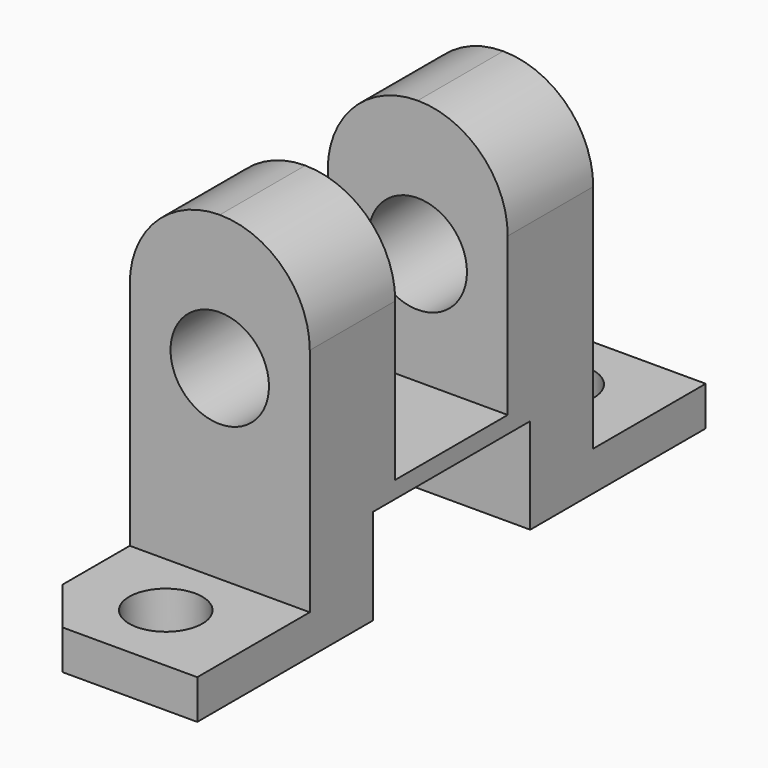
from build123d import *

# Parameters (mm, degrees)
F0_W      = 32
F0_H      = 113
F1_DEPTH  = 20
F2_W      = 32
F2_H      = 25
F3_DEPTH  = 13
F4_W      = 32
F4_H      = 35
F5_DEPTH  = 17
F6_W      = 32
F6_H      = 19
F7_DEPTH  = 44
F8_R      = 16
F9_R      = 15.99999
F10_R     = 16
F11_R     = 15.99999
F12_R     = 6.5
F13_DEPTH = 13
F14_R     = 6.5
F15_DEPTH = 13
F17_DEPTH = 25
F19_DEPTH = 25
F20_R     = 8.75
F21_DEPTH = 100


# Not quite as in the source:
# - a fillet or chamfer is up to 0.001 mm smaller than in the source, because OpenCascade refuses the exact size


with BuildPart() as f1:
    # F0 (on Top) → F1 (new body)
    with BuildSketch(Plane.XY):
        with Locations((-23.4775710851, 33.1401875504)):
            Rectangle(F0_W, F0_H)
    extrude(amount=F1_DEPTH)

    # F2 (on face) → F3 (cut)
    with BuildSketch(Plane.XY.offset(20)):
        with Locations((-23.4775710851, 77.1401875504)):
            Rectangle(F2_W, F2_H)
        with Locations((-23.4775710851, -10.8598124496)):
            Rectangle(F2_W, F2_H)
    extrude(amount=-F3_DEPTH, mode=Mode.SUBTRACT)

    # F4 (on face) → F5 (cut)
    with BuildSketch(Plane(origin=(0, 0, 0), x_dir=(1, 0, 0), z_dir=(0, 0, -1))):
        with Locations((-23.4775710851, -33.1401875504)):
            Rectangle(F4_W, F4_H)
    extrude(amount=-F5_DEPTH, mode=Mode.SUBTRACT)

    # F6 (on face) → F7 (join)
    with BuildSketch(Plane.XY.offset(20)):
        with Locations((-23.4775710851, 55.1401875504)):
            Rectangle(F6_W, F6_H)
        with Locations((-23.4775710851, 11.1401875504)):
            Rectangle(F6_W, F6_H)
    extrude(amount=F7_DEPTH)

    # F8
    f8_edges = [f1.edges().sort_by_distance(p)[0] for p in [
        (-39.477571, 55.140188, 64),
    ]]
    fillet(f8_edges, radius=F8_R)

    # F9 (radius 16 in the source; OpenCascade refuses exactly that, so slightly less here)
    f9_edges = [f1.edges().sort_by_distance(p)[0] for p in [
        (-7.477571, 55.140188, 64),
    ]]
    fillet(f9_edges, radius=F9_R)

    # F10
    f10_edges = [f1.edges().sort_by_distance(p)[0] for p in [
        (-39.477571, 11.140188, 64),
    ]]
    fillet(f10_edges, radius=F10_R)

    # F11 (radius 16 in the source; OpenCascade refuses exactly that, so slightly less here)
    f11_edges = [f1.edges().sort_by_distance(p)[0] for p in [
        (-7.477571, 11.140188, 64),
    ]]
    fillet(f11_edges, radius=F11_R)

    # F12 (on face) → F13 (cut)
    with BuildSketch(Plane.XY.offset(7)):
        with Locations((-23.4775710851, -10.3598124496)):
            Circle(F12_R)
    extrude(amount=-F13_DEPTH, mode=Mode.SUBTRACT)

    # F14 (on face) → F15 (cut)
    with BuildSketch(Plane.XY.offset(7)):
        with Locations((-23.4775710851, 76.6401875504)):
            Circle(F14_R)
    extrude(amount=-F15_DEPTH, mode=Mode.SUBTRACT)

    # F16 (on face) → F17 (cut)
    with BuildSketch(Plane.XY.offset(7)):
        Polygon((-39.4775710851, -13.3598124496), (-39.4775710851, -23.3598124496), (-31.4775710851, -23.3598124496), align=None)
    extrude(amount=-F17_DEPTH, mode=Mode.SUBTRACT)

    # F18 (on face) → F19 (cut)
    with BuildSketch(Plane.XY.offset(7)):
        Polygon((-31.4775710851, 89.6401875504), (-39.4775710851, 89.6401875504), (-39.4775710851, 79.6401875504), align=None)
    extrude(amount=-F19_DEPTH, mode=Mode.SUBTRACT)

    # F20 (on face) → F21 (cut)
    with BuildSketch(Plane.XZ.offset(-1.6401875504)):
        with Locations((-23.4775710851, 40)):
            Circle(F20_R)
    extrude(amount=-F21_DEPTH, mode=Mode.SUBTRACT)


solid = f1.part
